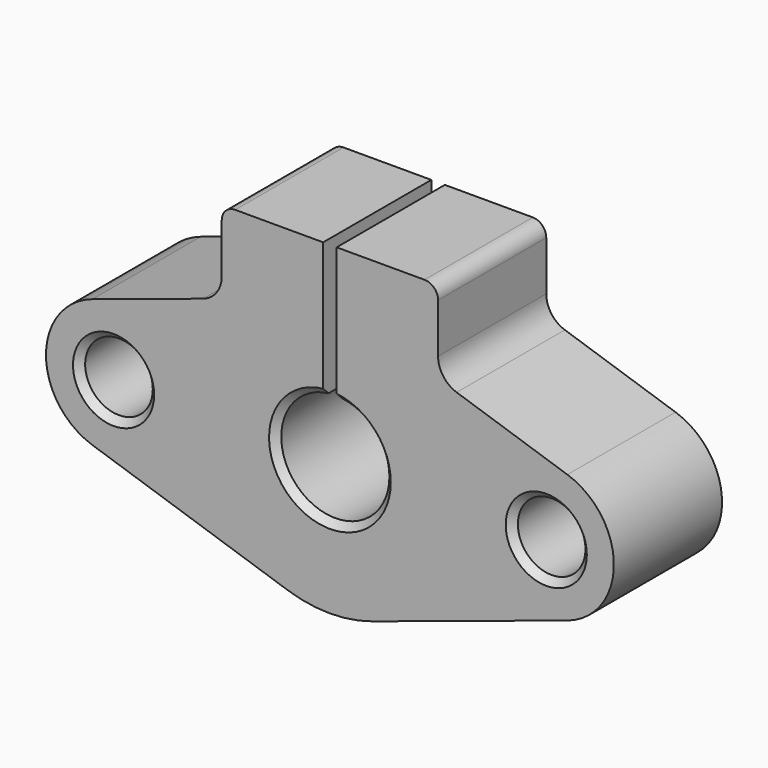
from build123d import *

# Parameters (mm, degrees)
F0_R     = 2.5
F1_DEPTH = 10
F2_SIZE  = 0.5


# Not quite as in the source:
# - a feature names something its author has since deleted; it is built from what else it names


with BuildPart() as f1:
    # F0 (on Front) → F1 (new body)
    with BuildSketch(Plane.XZ):
        with BuildLine():
            Line((0.5, 14), (0.5, 9.9874921777))
            ThreePointArc((0.5, 9.9874921777), (7.2456883731, 6.892024376), (10, 0))
            ThreePointArc((10, 0), (8.100925873, -5.8630196998), (3.125, -9.499177596))
            Line((3.125, -9.499177596), (17.5625, -4.749588798))
            ThreePointArc((17.5625, -4.749588798), (11, 0), (17.5625, 4.749588798))
            Line((17.5625, 4.749588798), (9.375, 7.4430785492))
            ThreePointArc((9.375, 7.4430785492), (8.3798148254, 8.1703101285), (8, 9.3429140684))
            Line((8, 9.3429140684), (8, 13))
            ThreePointArc((8, 13), (7.7071067812, 13.7071067812), (7, 14))
            Line((7, 14), (0.5, 14))
        make_face()
        with BuildLine():
            ThreePointArc((17.5625, 4.749588798), (11, 0), (17.5625, -4.749588798))
            ThreePointArc((17.5625, -4.749588798), (20.0504629365, -2.9315098499), (21, 0))
            ThreePointArc((21, 0), (20.0504629365, 2.9315098499), (17.5625, 4.749588798))
        make_face()
        with Locations((16, 0)):
            Circle(F0_R, mode=Mode.SUBTRACT)
        with BuildLine():
            ThreePointArc((-3.125, -9.499177596), (-9.9104859097, 1.3350164915), (-0.5, 9.9874921777))
            Line((-0.5, 9.9874921777), (-0.5, 14))
            Line((-0.5, 14), (-7, 14))
            ThreePointArc((-7, 14), (-7.7071067812, 13.7071067812), (-8, 13))
            Line((-8, 13), (-8, 9.3429140684))
            ThreePointArc((-8, 9.3429140684), (-8.3798148254, 8.1703101285), (-9.375, 7.4430785492))
            Line((-9.375, 7.4430785492), (-17.5625, 4.749588798))
            ThreePointArc((-17.5625, 4.749588798), (-13.0684901501, 4.0504629365), (-11, 0))
            ThreePointArc((-11, 0), (-13.0684901501, -4.0504629365), (-17.5625, -4.749588798))
            Line((-17.5625, -4.749588798), (-3.125, -9.499177596))
        make_face()
        with BuildLine():
            ThreePointArc((-17.5625, 4.749588798), (-21, 0), (-17.5625, -4.749588798))
            ThreePointArc((-17.5625, -4.749588798), (-13.0684901501, -4.0504629365), (-11, 0))
            ThreePointArc((-11, 0), (-13.0684901501, 4.0504629365), (-17.5625, 4.749588798))
        make_face()
        with Locations((-16, 0)):
            Circle(F0_R, mode=Mode.SUBTRACT)
        with BuildLine():
            ThreePointArc((0.5, 3.9686269666), (3, 2.6457513111), (4, 0))
            ThreePointArc((4, 0), (-2.6457513111, -3), (-0.5, 3.9686269666))
            Line((-0.5, 3.9686269666), (-0.5, 9.9874921777))
            ThreePointArc((-0.5, 9.9874921777), (-9.9104859097, 1.3350164915), (-3.125, -9.499177596))
            ThreePointArc((-3.125, -9.499177596), (0, -10), (3.125, -9.499177596))
            ThreePointArc((3.125, -9.499177596), (8.100925873, -5.8630196998), (10, 0))
            ThreePointArc((10, 0), (7.2456883731, 6.892024376), (0.5, 9.9874921777))
            Line((0.5, 9.9874921777), (0.5, 3.9686269666))
        make_face()
    extrude(amount=F1_DEPTH)

    # F2
    f2_edges = [f1.edges().sort_by_distance(p)[0] for p in [
        (-18.5, -10, 0),
        (0, -10, -4),
        (13.5, -10, 0),
        (13.5, 0, 0),
        (0, 0, -4),
        (-18.5, 0, 0),
    ]]
    chamfer(f2_edges, length=F2_SIZE)


solid = f1.part
